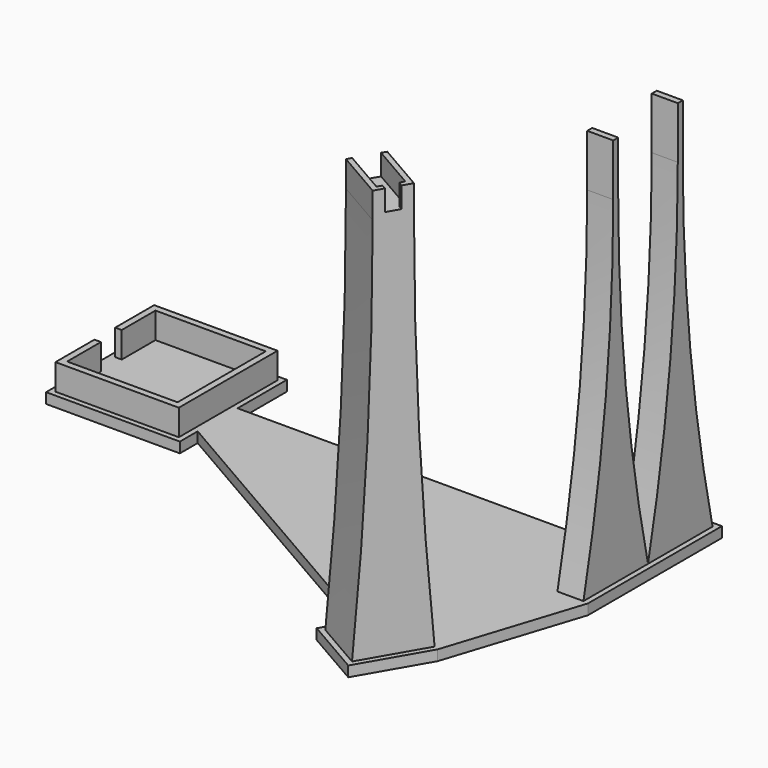
from build123d import *

# Parameters (mm, degrees)
F1_DEPTH  = 10
F5_DEPTH  = 10
F4_W      = 1.2
F4_H      = 20
F12_DEPTH = 8
F13_W     = 22
F13_H     = 13.3
F14_DEPTH = 2
F17_DEPTH = 22
F19_ANGLE = -30
F21_DEPTH = 4


# Not quite as in the source:
# - the program builds the solid bodies; features that only make, move or delete a surface that nothing else refers to are left out


with BuildPart() as f1:
    # F0 (on Top) → F1 (new body)
    with BuildSketch(Plane.XY):
        Polygon((-21.2, 21.2), (21.2, 21.2), (21.2, -21.2), (-21.2, -21.2), (-21.2, -5), (-23.7, -5), (-23.7, -23.7), (23.7, -23.7), (23.7, 23.7), (-23.7, 23.7), (-23.7, 5), (-21.2, 5), align=None)
    extrude(amount=F1_DEPTH)



with BuildPart() as f5:
    # F4 (on line) → F5 (new body)
    with BuildSketch(Plane.YZ.offset(175)):
        with BuildLine():
            Line((15.5, 130), (15.5, 0))
            Line((15.5, 0), (31, 0))
            ThreePointArc((31, 0), (20.2857494387, 64.6079324383), (16.7, 130))
            Line((16.7, 130), (16.7, 150))
            Line((16.7, 150), (15.5, 150))
            Line((15.5, 150), (15.5, 130))
        make_face()
        with BuildLine():
            ThreePointArc((14.3, 130), (10.7142505613, 64.6079324383), (0, 0))
            Line((0, 0), (15.5, 0))
            Line((15.5, 0), (15.5, 130))
            Line((15.5, 130), (15.5, 150))
            Line((15.5, 150), (14.3, 150))
            Line((14.3, 150), (14.3, 130))
        make_face()
    extrude(amount=F5_DEPTH)

    # F4 (on line) → F5, piece 2 (join)
    with BuildSketch(Plane.YZ.offset(175)):
        with BuildLine():
            Line((-15.5, 0), (0, 0))
            ThreePointArc((0, 0), (-10.7142505613, 64.6079324383), (-14.3, 130))
            Line((-14.3, 130), (-15.5, 130))
            Line((-15.5, 130), (-15.5, 0))
        make_face()
        with BuildLine():
            Line((-31, 0), (-15.5, 0))
            Line((-15.5, 0), (-15.5, 130))
            Line((-15.5, 130), (-16.7, 130))
            ThreePointArc((-16.7, 130), (-20.2857494387, 64.6079324383), (-31, 0))
        make_face()
        with Locations((-14.9, 140)):
            Rectangle(F4_W, F4_H)
        with Locations((-16.1, 140)):
            Rectangle(F4_W, F4_H)
    extrude(amount=F5_DEPTH)


with BuildPart() as f12:
    # F11 (on line) → F12 (new body)
    with BuildSketch(Plane.XY.offset(150)):
        Polygon((141.5544456623, -82.85), (161.5544456623, -82.85), (161.5544456623, -84.8), (163.5544456623, -84.8), (163.5544456623, -80.85), (141.5544456623, -80.85), align=None)
    extrude(amount=F12_DEPTH)



with BuildPart() as f12b:
    # F11 (on line) → F12, piece 2 (new body)
    with BuildSketch(Plane.XY.offset(150)):
        Polygon((161.5544456623, -92.15), (141.5544456623, -92.15), (141.5544456623, -94.15), (163.5544456623, -94.15), (163.5544456623, -90.2), (161.5544456623, -90.2), align=None)
    extrude(amount=F12_DEPTH)


with BuildPart() as f12_1:
    add(f12.part)

    add(f12b.part)  # F14 merges F12b
    # F13 (on line) → F14 (join)
    with BuildSketch(Plane.XY.offset(150)):
        with Locations((152.5544456623, -87.5)):
            Rectangle(F13_W, F13_H)
    extrude(amount=-F14_DEPTH)

    # F16 (on face) → F17 (join)
    with BuildSketch(Plane(origin=(163.5544456623, 0, 0), x_dir=(0, -1, 0), z_dir=(-1, 0, 0))):
        with BuildLine():
            Line((87.5, 0), (87.5, 148))
            Line((87.5, 148), (80.85, 148))
            ThreePointArc((80.85, 148), (79.1866617309, 73.9253374966), (74.2, 0))
            Line((74.2, 0), (87.5, 0))
        make_face()
        with BuildLine():
            Line((94.15, 148), (87.5, 148))
            Line((87.5, 148), (87.5, 0))
            Line((87.5, 0), (100.8, 0))
            ThreePointArc((100.8, 0), (95.8133382691, 73.9253374966), (94.15, 148))
        make_face()
    extrude(amount=F17_DEPTH)

    # F18: union 


with BuildPart() as f12_2:
    # F19: moved
    add(f12_1.part.rotate(Axis((151.5544456623, -87.5, 75), (0, 0, 1)), F19_ANGLE))


with BuildPart() as f1_1:
    add(f1.part)

    add(f5.part)  # F21 merges F5

    add(f12_2.part)  # F21 merges F12
    # F20 (on Top) → F21 (join)
    with BuildSketch(Plane.XY):
        Polygon((-25.7, 25.7), (-25.7, -25.7), (25.7, -25.7), (25.7, -17.1473029949), (140.1621408169, -83.2320508076), (133.5121408169, -94.7501886779), (156.0288013153, -107.7501886779), (170.4353579421, -82.7973006382), (187, -31.313824878), (187, 0), (187, 33), (173, 33), (173, 2), (25.7, 2), (25.7, 25.7), align=None)
        Polygon((23.7, 0), (175, 0), (175, 31), (185, 31), (185, 0), (185, -31), (168.5967505077, -81.9818621297), (155.2967505077, -105.0181378703), (136.2441916244, -94.0181378703), (142.8941916244, -82.5), (23.7, -13.6832013798), (23.7, -23.7), (-23.7, -23.7), (-23.7, 23.7), (23.7, 23.7), align=None, mode=Mode.SUBTRACT)
        Polygon((175, 31), (175, 0), (23.7, 0), (23.7, 23.7), (-23.7, 23.7), (-23.7, -23.7), (23.7, -23.7), (23.7, -13.6832013798), (142.8941916244, -82.5), (136.2441916244, -94.0181378703), (155.2967505077, -105.0181378703), (168.5967505077, -81.9818621297), (185, -31), (185, 0), (185, 31), align=None)
    extrude(amount=-F21_DEPTH)


solid = f1_1.part
